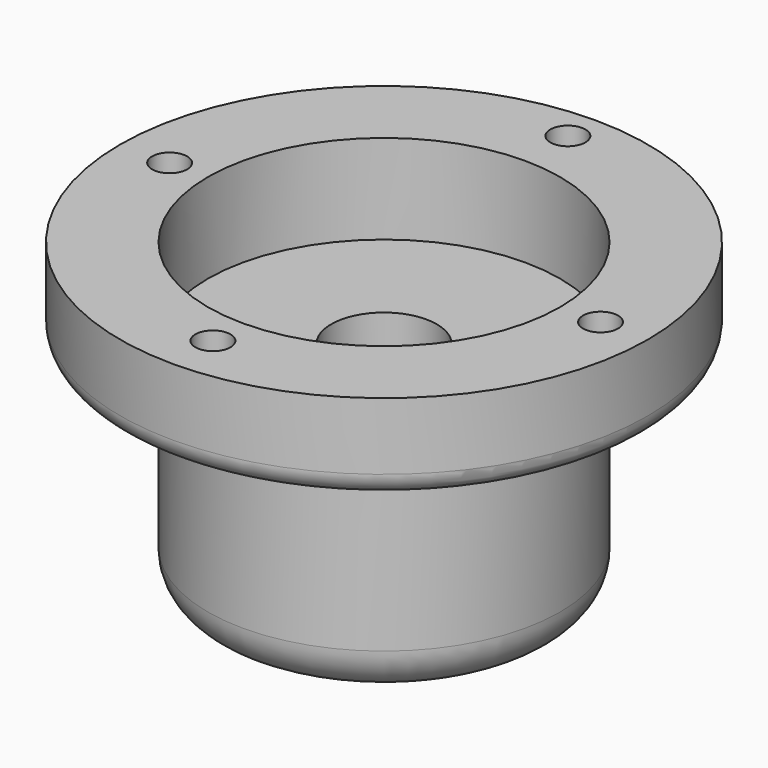
from build123d import *

# Parameters (mm, degrees)
F0_R     = 19.99996
F0_R_2   = 5.9944
F1_DEPTH = 25.4
F0_R_3   = 29.972
F0_R_4   = 1.9939
F2_DEPTH = 10.16
F3_R     = 5.08


# Not quite as in the source:
# - a fillet or chamfer that OpenCascade refuses, or shapes differently, is made with other operations: its cross-section is extruded or revolved along the edge and cut away or added
# - a feature names something its author has since deleted; it is built from what else it names


with BuildPart() as f1:
    # F0 (on Top) → F1 (new body)
    with BuildSketch(Plane.XY):
        Circle(F0_R)
        Circle(F0_R_2, mode=Mode.SUBTRACT)
    extrude(amount=-F1_DEPTH)

    # F3
    f3_edges = [f1.edges().sort_by_distance(p)[0] for p in [
        (-19.99996, 0, -25.4),
    ]]
    fillet(f3_edges, radius=F3_R)


with BuildPart() as f2:
    # F0 (on Top) → F2 (new body)
    with BuildSketch(Plane.XY):
        Circle(F0_R_3)
        with Locations((0, -24.2790300399)):
            Circle(F0_R_4, mode=Mode.SUBTRACT)
        with Locations((-24.3405103683, 0)):
            Circle(F0_R_4, mode=Mode.SUBTRACT)
        Circle(F0_R, mode=Mode.SUBTRACT)
        with Locations((24.5888829231, 0)):
            Circle(F0_R_4, mode=Mode.SUBTRACT)
        with Locations((0, 26.0943584144)):
            Circle(F0_R_4, mode=Mode.SUBTRACT)
    extrude(amount=F2_DEPTH)

    # F4: fillet of radius 2.54 on 1 edges, made by hand

    # F4_s1 → F4_t2 (revolve, cut)
    with BuildSketch(Plane.XZ):
        with BuildLine():
            ThreePointArc((29.972, 2.54), (29.2280512242, 0.7439487758), (27.432, 0))
            Line((27.432, 0), (29.972, 0))
            Line((29.972, 0), (29.972, 2.54))
        make_face()
    revolve(axis=Axis((0, 0, 0), (0, 0, 1)), mode=Mode.SUBTRACT)


solid = Compound([f1.part, f2.part])
